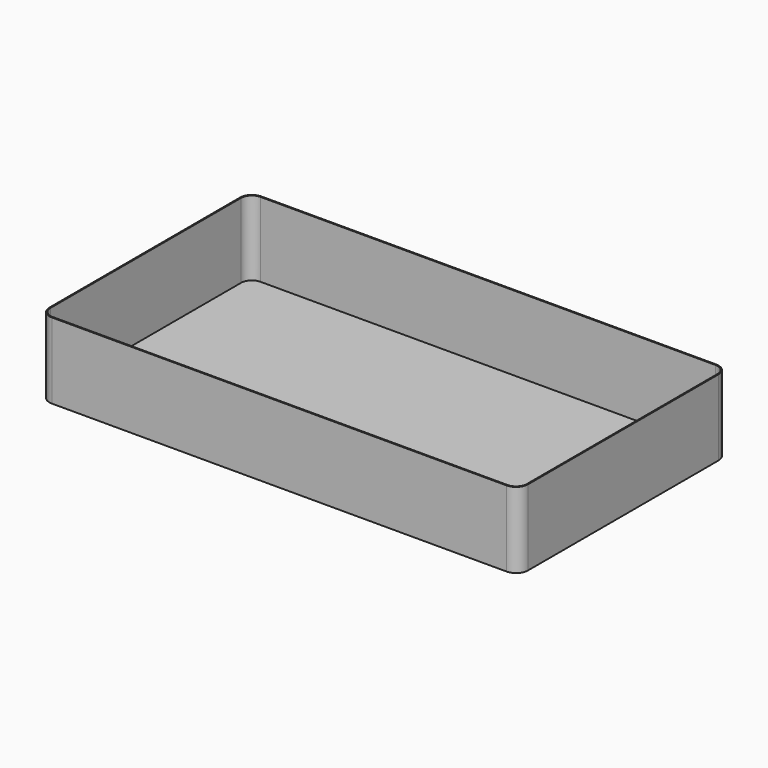
from build123d import *

# Parameters (mm, degrees)
F1_DEPTH = 0.5
F2_DEPTH = 35


with BuildPart() as f1:
    # F0 (on Top) → F1 (new body)
    with BuildSketch(Plane.XY):
        with BuildLine():
            Line((110.5, -55), (110.5, 55))
            ThreePointArc((110.5, 55), (108.8890872965, 58.8890872965), (105, 60.5))
            Line((105, 60.5), (-105, 60.5))
            ThreePointArc((-105, 60.5), (-108.8890872965, 58.8890872965), (-110.5, 55))
            Line((-110.5, 55), (-110.5, -55))
            ThreePointArc((-110.5, -55), (-108.8890872965, -58.8890872965), (-105, -60.5))
            Line((-105, -60.5), (105, -60.5))
            ThreePointArc((105, -60.5), (108.8890872965, -58.8890872965), (110.5, -55))
        make_face()
        with BuildLine():
            ThreePointArc((110, -55), (108.5355339059, -58.5355339059), (105, -60))
            Line((105, -60), (-105, -60))
            ThreePointArc((-105, -60), (-108.5355339059, -58.5355339059), (-110, -55))
            Line((-110, -55), (-110, 55))
            ThreePointArc((-110, 55), (-108.5355339059, 58.5355339059), (-105, 60))
            Line((-105, 60), (105, 60))
            ThreePointArc((105, 60), (108.5355339059, 58.5355339059), (110, 55))
            Line((110, 55), (110, -55))
        make_face(mode=Mode.SUBTRACT)
        with BuildLine():
            Line((-105, -60), (105, -60))
            ThreePointArc((105, -60), (108.5355339059, -58.5355339059), (110, -55))
            Line((110, -55), (110, 55))
            ThreePointArc((110, 55), (108.5355339059, 58.5355339059), (105, 60))
            Line((105, 60), (-105, 60))
            ThreePointArc((-105, 60), (-108.5355339059, 58.5355339059), (-110, 55))
            Line((-110, 55), (-110, -55))
            ThreePointArc((-110, -55), (-108.5355339059, -58.5355339059), (-105, -60))
        make_face()
    extrude(amount=F1_DEPTH)

    # F0 (on Top) → F2 (join)
    with BuildSketch(Plane.XY):
        with BuildLine():
            Line((110.5, -55), (110.5, 55))
            ThreePointArc((110.5, 55), (108.8890872965, 58.8890872965), (105, 60.5))
            Line((105, 60.5), (-105, 60.5))
            ThreePointArc((-105, 60.5), (-108.8890872965, 58.8890872965), (-110.5, 55))
            Line((-110.5, 55), (-110.5, -55))
            ThreePointArc((-110.5, -55), (-108.8890872965, -58.8890872965), (-105, -60.5))
            Line((-105, -60.5), (105, -60.5))
            ThreePointArc((105, -60.5), (108.8890872965, -58.8890872965), (110.5, -55))
        make_face()
        with BuildLine():
            ThreePointArc((110, -55), (108.5355339059, -58.5355339059), (105, -60))
            Line((105, -60), (-105, -60))
            ThreePointArc((-105, -60), (-108.5355339059, -58.5355339059), (-110, -55))
            Line((-110, -55), (-110, 55))
            ThreePointArc((-110, 55), (-108.5355339059, 58.5355339059), (-105, 60))
            Line((-105, 60), (105, 60))
            ThreePointArc((105, 60), (108.5355339059, 58.5355339059), (110, 55))
            Line((110, 55), (110, -55))
        make_face(mode=Mode.SUBTRACT)
    extrude(amount=F2_DEPTH)


solid = f1.part
